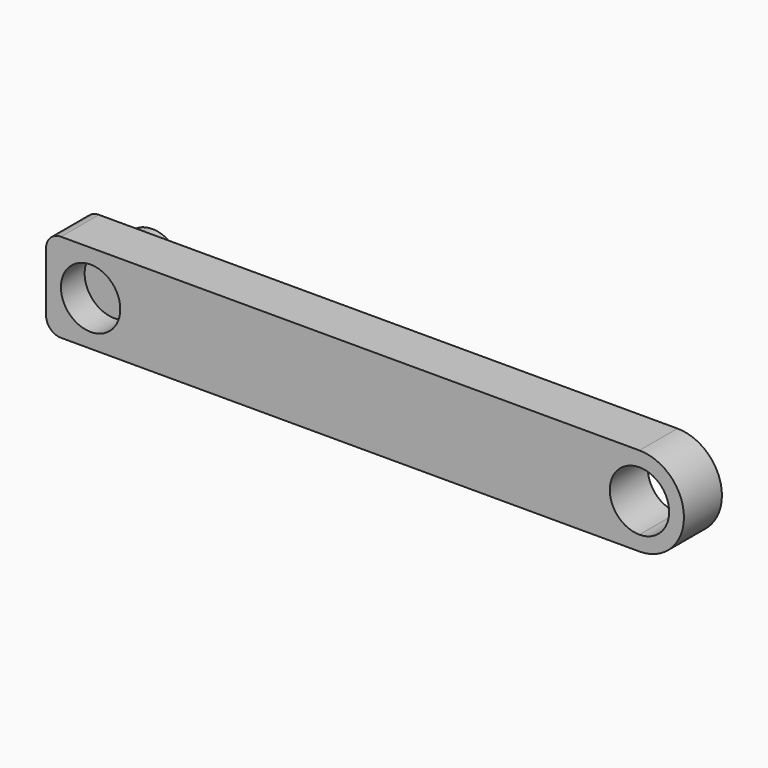
from build123d import *

# Parameters (mm, degrees)
F1_DEPTH = 8
F2_R     = 2.5
F3_R     = 5
F4_DEPTH = 5
F5_R     = 5
F6_DEPTH = 5


# Not quite as in the source:
# - a feature names something its author has since deleted; it is built from what else it names


with BuildPart() as f1:
    # F0 (on Front) → F1 (new body)
    with BuildSketch(Plane.XZ):
        with BuildLine():
            ThreePointArc((0, -7.5), (-7.5, 0), (0, 7.5))
            Line((0, 7.5), (-100, 7.5))
            Line((-100, 7.5), (-100, -7.5))
            Line((-100, -7.5), (0, -7.5))
        make_face()
        with BuildLine():
            Line((0, 5), (0, 7.5))
            ThreePointArc((0, 7.5), (-7.5, 0), (0, -7.5))
            Line((0, -7.5), (0, -5))
            ThreePointArc((0, -5), (-5, 0), (0, 5))
        make_face()
        with BuildLine():
            ThreePointArc((0, -7.5), (5.3033008589, -5.3033008589), (7.5, 0))
            ThreePointArc((7.5, 0), (5.3033008589, 5.3033008589), (0, 7.5))
            Line((0, 7.5), (0, 5))
            ThreePointArc((0, 5), (3.5355339059, 3.5355339059), (5, 0))
            ThreePointArc((5, 0), (3.5355339059, -3.5355339059), (0, -5))
            Line((0, -5), (0, -7.5))
        make_face()
    extrude(amount=F1_DEPTH)

    # F2
    f2_edges = [f1.edges().sort_by_distance(p)[0] for p in [
        (-100, -4, 7.5),
        (-100, -4, -7.5),
    ]]
    fillet(f2_edges, radius=F2_R)

    # F3 (on face) → F4 (join)
    with BuildSketch(Plane(origin=(0, 0, 0), x_dir=(-1, 0, 0), z_dir=(0, 1, 0))):
        with Locations((92.5, 0)):
            Circle(F3_R)
    extrude(amount=F4_DEPTH)

    # F5 (on face) → F6 (cut)
    with BuildSketch(Plane.XZ.offset(8)):
        with Locations((-92.5, 0)):
            Circle(F5_R)
    extrude(amount=-F6_DEPTH, mode=Mode.SUBTRACT)


solid = f1.part
